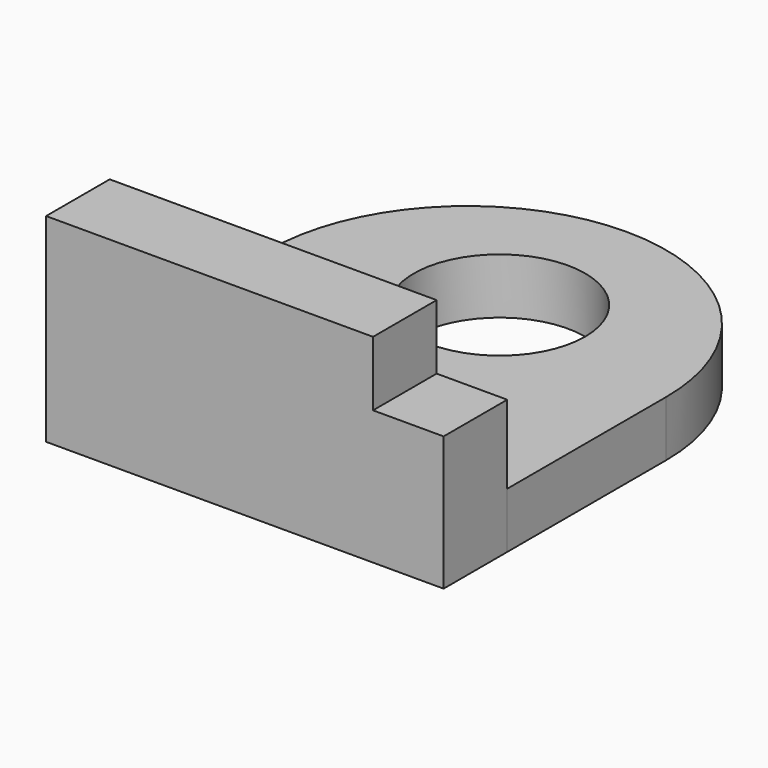
from build123d import *

# Parameters (mm, degrees)
F0_W     = 127
F0_H     = 63.5
F1_DEPTH = 25.4
F2_W     = 22.5477049351
F2_H     = 20.6739342883
F3_DEPTH = 25.4
F4_W     = 127
F4_H     = 17.7800003439
F5_DEPTH = 127
F6_R     = 63.5
F7_R     = 63.49999
F8_R     = 27.3600762243
F9_DEPTH = 25.4


# Not quite as in the source:
# - a fillet or chamfer is up to 0.001 mm smaller than in the source, because OpenCascade refuses the exact size


with BuildPart() as f1:
    # F0 (on Front) → F1 (new body)
    with BuildSketch(Plane.XZ):
        Rectangle(F0_W, F0_H)
    extrude(amount=F1_DEPTH)

    # F2 (on face) → F3 (cut)
    with BuildSketch(Plane.XZ.offset(25.4)):
        with Locations((52.2261475325, 21.4130328558)):
            Rectangle(F2_W, F2_H)
    extrude(amount=-F3_DEPTH, mode=Mode.SUBTRACT)


with BuildPart() as f5:
    # F4 (on Front) → F5 (new body)
    with BuildSketch(Plane.XZ):
        with Locations((0, -22.859999828)):
            Rectangle(F4_W, F4_H)
    extrude(amount=-F5_DEPTH)

    # F6
    f6_edges = [f5.edges().sort_by_distance(p)[0] for p in [
        (63.5, 127, -22.86),
    ]]
    fillet(f6_edges, radius=F6_R)

    # F7 (radius 63.5 in the source; OpenCascade refuses exactly that, so slightly less here)
    f7_edges = [f5.edges().sort_by_distance(p)[0] for p in [
        (-63.5, 127, -22.86),
    ]]
    fillet(f7_edges, radius=F7_R)

    # F8 (on face) → F9 (cut)
    with BuildSketch(Plane.XY.offset(-13.9699996561)):
        with Locations((0, 76.3110369444)):
            Circle(F8_R)
    extrude(amount=-F9_DEPTH, mode=Mode.SUBTRACT)


solid = Compound([f1.part, f5.part])
